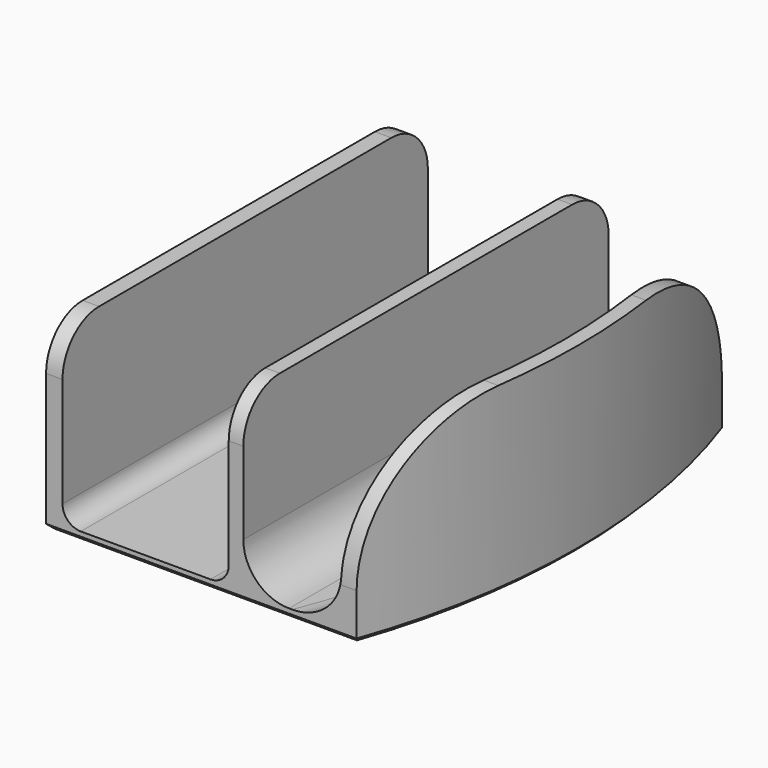
from build123d import *

# Parameters (mm, degrees)
F0_W         = 1.8
F0_H         = 50
F0_W_2       = 18.2
F0_W_3       = 1.6
F1_DEPTH     = 1
F2_DEPTH     = 20
F3_DEPTH     = 20
F4_T4_DEPTH  = 76.7042031505
F4_T9_DEPTH  = 76.6048284538
F4_T14_DEPTH = 76.8048284538
F4_T19_DEPTH = 76.7042031505
F4_T24_DEPTH = 76.6048284538
F4_T29_DEPTH = 76.8048284538
F5_R         = 5
F6_R         = 2
F7_R         = 5
F8_SIZE      = 0.5


# Not quite as in the source:
# - a fillet or chamfer that OpenCascade refuses, or shapes differently, is made with other operations: its cross-section is extruded or revolved along the edge and cut away or added


with BuildPart() as f1:
    # F0 (on Top) → F1 (new body)
    with BuildSketch(Plane.XY):
        with Locations((0.9, 25)):
            Rectangle(F0_W, F0_H)
        with Locations((10.9, 25)):
            Rectangle(F0_W_2, F0_H)
        with Locations((20.8, 25)):
            Rectangle(F0_W_3, F0_H)
        with BuildLine():
            Line((21.6, 50), (21.6, 0))
            Line((21.6, 0), (32.3006253033, 0))
            ThreePointArc((32.3006253033, 0), (36.6893218813, 25), (32.3006253033, 50))
            Line((32.3006253033, 50), (21.6, 50))
        make_face()
        with BuildLine():
            ThreePointArc((32.3006253033, 50), (36.6893218813, 25), (32.3006253033, 0))
            Line((32.3006253033, 0), (34, 0))
            ThreePointArc((34, 0), (38.2893218813, 25), (34, 50))
            Line((34, 50), (32.3006253033, 50))
        make_face()
    extrude(amount=F1_DEPTH)

    # F0 (on Top) → F2 (join)
    with BuildSketch(Plane.XY):
        with Locations((0.9, 25)):
            Rectangle(F0_W, F0_H)
        with Locations((20.8, 25)):
            Rectangle(F0_W_3, F0_H)
    extrude(amount=F2_DEPTH)

    # F0 (on Top) → F3 (join)
    with BuildSketch(Plane.XY):
        with BuildLine():
            ThreePointArc((32.3006253033, 50), (36.6893218813, 25), (32.3006253033, 0))
            Line((32.3006253033, 0), (34, 0))
            ThreePointArc((34, 0), (38.2893218813, 25), (34, 50))
            Line((34, 50), (32.3006253033, 50))
        make_face()
    extrude(amount=F3_DEPTH)

    # F4: fillet of radius 15 on 6 edges, made by hand


with BuildPart() as f4_tool2:
    # F4_s3 → F4_t4 (new body)
    with BuildSketch(Plane.YZ.offset(-5.2017889236)):
        with BuildLine():
            ThreePointArc((15.0009656854, 20.0004), (4.3933982822, 15.6066017178), (-0.0004, 4.9990343146))
            Line((-0.0004, 4.9990343146), (-1.5005365685, 4.9990343146))
            ThreePointArc((-1.5005365685, 4.9990343146), (-1.5001365685, 12.4995171573), (-1.5001365685, 20))
            Line((-1.5001365685, 20), (0, 21.5001365685))
            ThreePointArc((0, 21.5001365685), (7.5004828427, 21.5001365685), (15.0009656854, 21.5005365685))
            Line((15.0009656854, 21.5005365685), (15.0009656854, 20.0004))
        make_face()
    extrude(amount=F4_T4_DEPTH)

    split(bisect_by=Plane.YZ.offset(21.6), keep=Keep.TOP)


with BuildPart() as f1_1:
    add(f1.part)

    # F4_t1: cut F4_tool2
    add(f4_tool2.part, mode=Mode.SUBTRACT)


with BuildPart() as f4_tool7:
    # F4_s8 → F4_t9 (new body)
    with BuildSketch(Plane.YZ.offset(-17.5024142269)):
        with BuildLine():
            ThreePointArc((15.0009656854, 20.0004), (4.3933982822, 15.6066017178), (-0.0004, 4.9990343146))
            Line((-0.0004, 4.9990343146), (-1.5005365685, 4.9990343146))
            ThreePointArc((-1.5005365685, 4.9990343146), (-1.5001365685, 12.4995171573), (-1.5001365685, 20))
            Line((-1.5001365685, 20), (0, 21.5001365685))
            ThreePointArc((0, 21.5001365685), (7.5004828427, 21.5001365685), (15.0009656854, 21.5005365685))
            Line((15.0009656854, 21.5005365685), (15.0009656854, 20.0004))
        make_face()
    extrude(amount=F4_T9_DEPTH)

    split(bisect_by=Plane.YZ.offset(21.6), keep=Keep.TOP)


with BuildPart() as f1_2:
    add(f1_1.part)

    # F4_t6: cut F4_tool7
    add(f4_tool7.part, mode=Mode.SUBTRACT)


with BuildPart() as f4_tool12:
    # F4_s13 → F4_t14 (new body)
    with BuildSketch(Plane.YZ.offset(-37.5024142269)):
        with BuildLine():
            ThreePointArc((-0.0004, 4.9990343146), (4.3933982822, 15.6066017178), (15.0009656854, 20.0004))
            Line((15.0009656854, 20.0004), (15.0009656854, 21.5005365685))
            ThreePointArc((15.0009656854, 21.5005365685), (7.5004828427, 21.5001365685), (0, 21.5001365685))
            Line((0, 21.5001365685), (-1.5001365685, 20))
            ThreePointArc((-1.5001365685, 20), (-1.5001365685, 12.4995171573), (-1.5005365685, 4.9990343146))
            Line((-1.5005365685, 4.9990343146), (-0.0004, 4.9990343146))
        make_face()
    extrude(amount=F4_T14_DEPTH)

    split(bisect_by=Plane.YZ.offset(21.6), keep=Keep.TOP)


with BuildPart() as f1_3:
    add(f1_2.part)

    # F4_t11: cut F4_tool12
    add(f4_tool12.part, mode=Mode.SUBTRACT)


with BuildPart() as f4_tool17:
    # F4_s18 → F4_t19 (new body)
    with BuildSketch(Plane.YZ.offset(71.5024142269)):
        with BuildLine():
            ThreePointArc((34.9990343146, 20.0004), (45.6066017178, 15.6066017178), (50.0004, 4.9990343146))
            Line((50.0004, 4.9990343146), (51.5005365685, 4.9990343146))
            ThreePointArc((51.5005365685, 4.9990343146), (51.5001365685, 12.4995171573), (51.5001365685, 20))
            Line((51.5001365685, 20), (50, 21.5001365685))
            ThreePointArc((50, 21.5001365685), (42.4995171573, 21.5001365685), (34.9990343146, 21.5005365685))
            Line((34.9990343146, 21.5005365685), (34.9990343146, 20.0004))
        make_face()
    extrude(amount=-F4_T19_DEPTH)

    split(bisect_by=Plane.YZ.offset(21.6), keep=Keep.TOP)


with BuildPart() as f1_4:
    add(f1_3.part)

    # F4_t16: cut F4_tool17
    add(f4_tool17.part, mode=Mode.SUBTRACT)


with BuildPart() as f4_tool22:
    # F4_s23 → F4_t24 (new body)
    with BuildSketch(Plane.YZ.offset(59.1024142269)):
        with BuildLine():
            ThreePointArc((34.9990343146, 20.0004), (45.6066017178, 15.6066017178), (50.0004, 4.9990343146))
            Line((50.0004, 4.9990343146), (51.5005365685, 4.9990343146))
            ThreePointArc((51.5005365685, 4.9990343146), (51.5001365685, 12.4995171573), (51.5001365685, 20))
            Line((51.5001365685, 20), (50, 21.5001365685))
            ThreePointArc((50, 21.5001365685), (42.4995171573, 21.5001365685), (34.9990343146, 21.5005365685))
            Line((34.9990343146, 21.5005365685), (34.9990343146, 20.0004))
        make_face()
    extrude(amount=-F4_T24_DEPTH)

    split(bisect_by=Plane.YZ.offset(21.6), keep=Keep.TOP)


with BuildPart() as f1_5:
    add(f1_4.part)

    # F4_t21: cut F4_tool22
    add(f4_tool22.part, mode=Mode.SUBTRACT)


with BuildPart() as f4_tool27:
    # F4_s28 → F4_t29 (new body)
    with BuildSketch(Plane.YZ.offset(39.3024142269)):
        with BuildLine():
            ThreePointArc((34.9990343146, 20.0004), (45.6066017178, 15.6066017178), (50.0004, 4.9990343146))
            Line((50.0004, 4.9990343146), (51.5005365685, 4.9990343146))
            ThreePointArc((51.5005365685, 4.9990343146), (51.5001365685, 12.4995171573), (51.5001365685, 20))
            Line((51.5001365685, 20), (50, 21.5001365685))
            ThreePointArc((50, 21.5001365685), (42.4995171573, 21.5001365685), (34.9990343146, 21.5005365685))
            Line((34.9990343146, 21.5005365685), (34.9990343146, 20.0004))
        make_face()
    extrude(amount=-F4_T29_DEPTH)

    split(bisect_by=Plane.YZ.offset(21.6), keep=Keep.TOP)


with BuildPart() as f1_6:
    add(f1_5.part)

    # F4_t26: cut F4_tool27
    add(f4_tool27.part, mode=Mode.SUBTRACT)

    # F5
    f5_edges = [f1_6.edges().sort_by_distance(p)[0] for p in [
        (36.689322, 25, 1),
        (21.6, 25, 1),
    ]]
    fillet(f5_edges, radius=F5_R)

    # F6
    f6_edges = [f1_6.edges().sort_by_distance(p)[0] for p in [
        (1.8, 25, 1),
        (20, 25, 1),
    ]]
    fillet(f6_edges, radius=F6_R)

    # F7
    f7_edges = [f1_6.edges().sort_by_distance(p)[0] for p in [
        (0.9, 0, 20),
        (20.8, 0, 20),
        (20.8, 50, 20),
        (0.9, 50, 20),
    ]]
    fillet(f7_edges, radius=F7_R)

    # F8
    f8_edges = [f1_6.edges().sort_by_distance(p)[0] for p in [
        (0, 25, 0),
        (17, 0, 0),
        (38.289322, 25, 0),
        (17, 50, 0),
    ]]
    chamfer(f8_edges, length=F8_SIZE)


solid = f1_6.part
